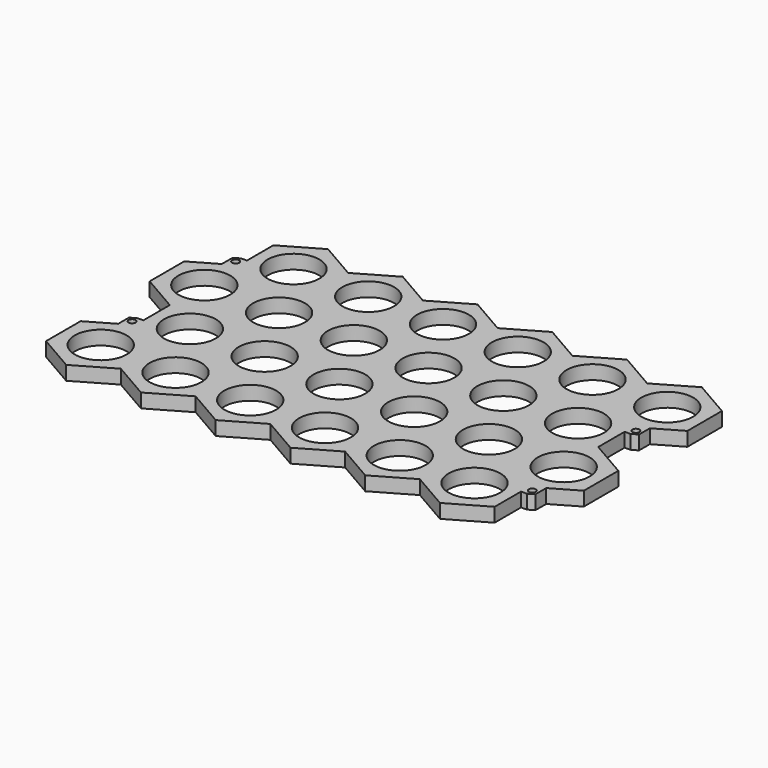
from build123d import *

# Parameters (mm, degrees)
F0_R     = 11.1
F0_R_2   = 1.5
F1_DEPTH = 6
F2_DEPTH = 6


# Not quite as in the source:
# - a feature names something its author has since deleted; it is built from what else it names


with BuildPart() as f1:
    # F0 (on Top) → F1 (new body)
    with BuildSketch(Plane.XY):
        Polygon((32, 18.4752086141), (16, 9.237604307), (16, -9.237604307), (32, -18.4752086141), (48, -9.237604307), (48, 9.237604307), align=None)
        with Locations((32, 0)):
            Circle(F0_R, mode=Mode.SUBTRACT)
        Polygon((16, -9.237604307), (16, 9.237604307), (0, 18.4752086141), (-2.5, 17.0318329411), (-5, 15.5884572681), (-16, 9.237604307), (-16, -9.237604307), (0, -18.4752086141), align=None)
        Circle(F0_R, mode=Mode.SUBTRACT)
        Polygon((0, 18.4752086141), (16, 9.237604307), (32, 18.4752086141), (32, 36.9504172281), (16, 46.1880215352), (0, 36.9504172281), (0, 22.805335633), (0, 21.36195996), align=None)
        with Locations((16, 27.7128129211)):
            Circle(F0_R, mode=Mode.SUBTRACT)
        Polygon((-2.5, 17.0318329411), (0, 18.4752086141), (0, 21.36195996), (-2.5, 22.805335633), (-5, 21.36195996), (-5, 18.4752086141), align=None)
        with Locations((-2.5, 19.918584287)):
            Circle(F0_R_2, mode=Mode.SUBTRACT)
        Polygon((32, 36.9504172281), (32, 18.4752086141), (48, 9.237604307), (64, 18.4752086141), (64, 36.9504172281), (48, 46.1880215352), align=None)
        with Locations((48, 27.7128129211)):
            Circle(F0_R, mode=Mode.SUBTRACT)
        Polygon((64, 18.4752086141), (48, 9.237604307), (48, -9.237604307), (64, -18.4752086141), (80, -9.237604307), (80, 9.237604307), align=None)
        with Locations((64, 0)):
            Circle(F0_R, mode=Mode.SUBTRACT)
        Polygon((16, 46.1880215352), (32, 36.9504172281), (48, 46.1880215352), (48, 64.6632301492), (32, 73.9008344563), (16, 64.6632301492), align=None)
        with Locations((32, 55.4256258422)):
            Circle(F0_R, mode=Mode.SUBTRACT)
        Polygon((64, 36.9504172281), (64, 18.4752086141), (80, 9.237604307), (96, 18.4752086141), (96, 36.9504172281), (80, 46.1880215352), align=None)
        with Locations((80, 27.7128129211)):
            Circle(F0_R, mode=Mode.SUBTRACT)
        Polygon((0, 36.9504172281), (16, 46.1880215352), (16, 64.6632301492), (0, 73.9008344563), (-2.5, 72.4574587833), (-5, 71.0140831103), (-16, 64.6632301492), (-16, 46.1880215352), align=None)
        with Locations((0, 55.4256258422)):
            Circle(F0_R, mode=Mode.SUBTRACT)
        Polygon((48, 64.6632301492), (48, 46.1880215352), (64, 36.9504172281), (80, 46.1880215352), (80, 64.6632301492), (64, 73.9008344563), align=None)
        with Locations((64, 55.4256258422)):
            Circle(F0_R, mode=Mode.SUBTRACT)
        Polygon((96, 18.4752086141), (80, 9.237604307), (80, -9.237604307), (96, -18.4752086141), (112, -9.237604307), (112, 9.237604307), align=None)
        with Locations((96, 0)):
            Circle(F0_R, mode=Mode.SUBTRACT)
        Polygon((32, 73.9008344563), (48, 64.6632301492), (64, 73.9008344563), (64, 92.3760430703), (48, 101.6136473774), (32, 92.3760430703), align=None)
        with Locations((48, 83.1384387633)):
            Circle(F0_R, mode=Mode.SUBTRACT)
        Polygon((96, 36.9504172281), (96, 18.4752086141), (112, 9.237604307), (128, 18.4752086141), (128, 36.9504172281), (112, 46.1880215352), align=None)
        with Locations((112, 27.7128129211)):
            Circle(F0_R, mode=Mode.SUBTRACT)
        Polygon((80, 64.6632301492), (80, 46.1880215352), (96, 36.9504172281), (112, 46.1880215352), (112, 64.6632301492), (96, 73.9008344563), align=None)
        with Locations((96, 55.4256258422)):
            Circle(F0_R, mode=Mode.SUBTRACT)
        Polygon((-2.5, 72.4574587833), (0, 73.9008344563), (0, 76.7875858022), (-2.5, 78.2309614752), (-5, 76.7875858022), (-5, 73.9008344563), align=None)
        with Locations((-2.5, 75.3442101292)):
            Circle(F0_R_2, mode=Mode.SUBTRACT)
        Polygon((64, 92.3760430703), (64, 73.9008344563), (80, 64.6632301492), (96, 73.9008344563), (96, 92.3760430703), (80, 101.6136473774), align=None)
        with Locations((80, 83.1384387633)):
            Circle(F0_R, mode=Mode.SUBTRACT)
        Polygon((128, 18.4752086141), (112, 9.237604307), (112, -9.237604307), (128, -18.4752086141), (144, -9.237604307), (144, 9.237604307), align=None)
        with Locations((128, 0)):
            Circle(F0_R, mode=Mode.SUBTRACT)
        Polygon((128, 36.9504172281), (128, 18.4752086141), (144, 9.237604307), (160, 18.4752086141), (160, 36.9504172281), (144, 46.1880215352), align=None)
        with Locations((144, 27.7128129211)):
            Circle(F0_R, mode=Mode.SUBTRACT)
        Polygon((112, 64.6632301492), (112, 46.1880215352), (128, 36.9504172281), (144, 46.1880215352), (144, 64.6632301492), (128, 73.9008344563), align=None)
        with Locations((128, 55.4256258422)):
            Circle(F0_R, mode=Mode.SUBTRACT)
        Polygon((96, 92.3760430703), (96, 73.9008344563), (112, 64.6632301492), (128, 73.9008344563), (128, 92.3760430703), (112, 101.6136473774), align=None)
        with Locations((112, 83.1384387633)):
            Circle(F0_R, mode=Mode.SUBTRACT)
        Polygon((160, 18.4752086141), (144, 9.237604307), (144, -9.237604307), (160, -18.4752086141), (176, -9.237604307), (176, 4.9074772881), (176, 6.3508529611), (176, 9.237604307), align=None)
        with Locations((160, 0)):
            Circle(F0_R, mode=Mode.SUBTRACT)
        Polygon((160, 36.9504172281), (160, 18.4752086141), (176, 9.237604307), (178.5, 10.68097998), (181, 12.124355653), (192, 18.4752086141), (192, 36.9504172281), (176, 46.1880215352), align=None)
        with Locations((176, 27.7128129211)):
            Circle(F0_R, mode=Mode.SUBTRACT)
        Polygon((144, 64.6632301492), (144, 46.1880215352), (160, 36.9504172281), (176, 46.1880215352), (176, 60.3331031303), (176, 61.7764788033), (176, 64.6632301492), (160, 73.9008344563), align=None)
        with Locations((160, 55.4256258422)):
            Circle(F0_R, mode=Mode.SUBTRACT)
        Polygon((128, 92.3760430703), (128, 73.9008344563), (144, 64.6632301492), (160, 73.9008344563), (160, 92.3760430703), (144, 101.6136473774), align=None)
        with Locations((144, 83.1384387633)):
            Circle(F0_R, mode=Mode.SUBTRACT)
        Polygon((160, 92.3760430703), (160, 73.9008344563), (176, 64.6632301492), (178.5, 66.1066058222), (181, 67.5499814952), (192, 73.9008344563), (192, 92.3760430703), (176, 101.6136473774), align=None)
        with Locations((176, 83.1384387633)):
            Circle(F0_R, mode=Mode.SUBTRACT)
    extrude(amount=F1_DEPTH)

    # F0 (on Top) → F2 (join)
    with BuildSketch(Plane.XY):
        Polygon((0, 18.4752086141), (16, 9.237604307), (32, 18.4752086141), (32, 36.9504172281), (16, 46.1880215352), (0, 36.9504172281), (0, 22.805335633), (0, 21.36195996), align=None)
        with Locations((16, 27.7128129211)):
            Circle(F0_R, mode=Mode.SUBTRACT)
        Polygon((0, 73.9008344563), (16, 64.6632301492), (32, 73.9008344563), (32, 92.3760430703), (16, 101.6136473774), (0, 92.3760430703), (0, 78.2309614752), (0, 76.7875858022), align=None)
        with Locations((16, 83.1384387633)):
            Circle(F0_R, mode=Mode.SUBTRACT)
        Polygon((178.5, 10.68097998), (176, 9.237604307), (176, 6.3508529611), (178.5, 4.9074772881), (181, 6.3508529611), (181, 9.237604307), align=None)
        with Locations((178.5, 7.7942286341)):
            Circle(F0_R_2, mode=Mode.SUBTRACT)
        Polygon((178.5, 66.1066058222), (176, 64.6632301492), (176, 61.7764788033), (178.5, 60.3331031303), (181, 61.7764788033), (181, 64.6632301492), align=None)
        with Locations((178.5, 63.2198544763)):
            Circle(F0_R_2, mode=Mode.SUBTRACT)
        Polygon((-5, 71.0140831103), (-2.5, 72.4574587833), (-5, 73.9008344563), align=None)
        Polygon((-2.5, 78.2309614752), (0, 76.7875858022), (0, 78.2309614752), align=None)
        Polygon((-2.5, 22.805335633), (0, 21.36195996), (0, 22.805335633), align=None)
        Polygon((-5, 15.5884572681), (-2.5, 17.0318329411), (-5, 18.4752086141), align=None)
        Polygon((176, 61.7764788033), (176, 60.3331031303), (178.5, 60.3331031303), align=None)
        Polygon((181, 67.5499814952), (178.5, 66.1066058222), (181, 64.6632301492), align=None)
        Polygon((178.5, 4.9074772881), (176, 6.3508529611), (176, 4.9074772881), align=None)
        Polygon((181, 12.124355653), (178.5, 10.68097998), (181, 9.237604307), align=None)
    extrude(amount=F2_DEPTH)


solid = f1.part
